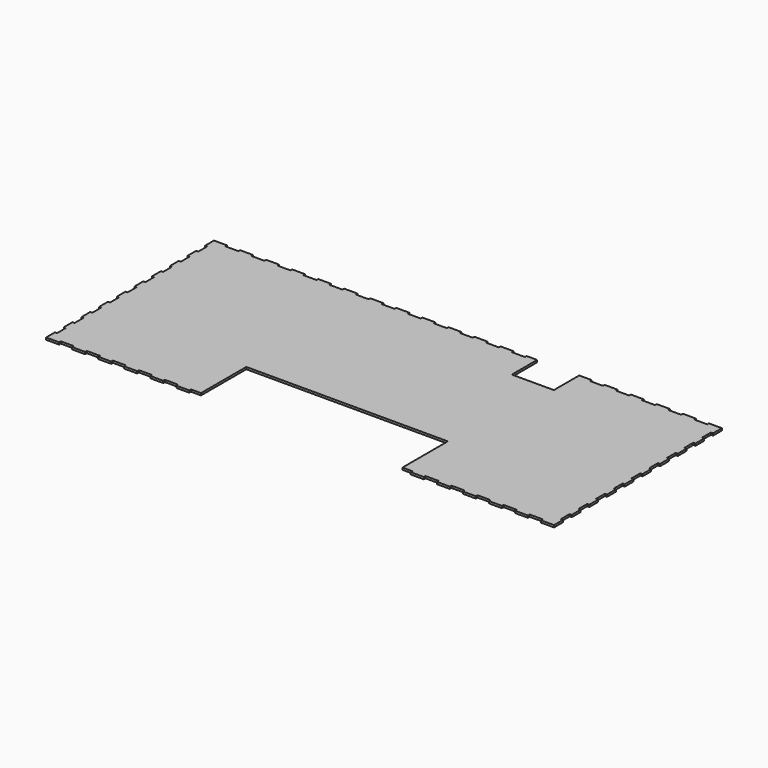
from build123d import *

# Parameters (mm, degrees)
F1_DEPTH = 3.175


# Not quite as in the source:
# - ends of sketch curves that miss each other by under 0.0002 mm in the source are joined
# - a feature names something its author has since deleted; it is built from what else it names


with BuildPart() as f1:
    # F0 (on Top) → F1 (new body)
    with BuildSketch(Plane.XY):
        Polygon((-364.473717838, 158.75), (-384.175, 158.75), (-384.175, 142.039473604), (-381, 142.039473604), (-381, 125.328947208), (-384.175, 125.328947208), (-384.175, 108.618420812), (-381, 108.618420812), (-381, 91.907894416), (-384.175, 91.907894416), (-384.175, 75.19736802), (-381, 75.19736802), (-381, 58.486841624), (-384.175, 58.486841624), (-384.175, 41.776315228), (-381, 41.776315228), (-381, 25.065788832), (-384.175, 25.065788832), (-384.175, 8.355262436), (-381, 8.355262436), (-381, -8.35526396), (-384.175, -8.35526396), (-384.175, -25.065790356), (-381, -25.065790356), (-381, -41.776316752), (-384.175, -41.776316752), (-384.175, -58.486843148), (-381, -58.486843148), (-381, -75.197369544), (-384.175, -75.197369544), (-384.175, -91.90789594), (-381, -91.90789594), (-381, -108.618422336), (-384.175, -108.618422336), (-384.175, -125.328948732), (-381, -125.328948732), (-381, -142.039475128), (-384.175, -142.039475128), (-384.175, -158.750001524), (-381, -158.750001524), (-364.473717838, -158.75), (-364.473717838, -155.575), (-344.772435676, -155.575), (-344.772435676, -158.75), (-325.071153514, -158.75), (-325.071153514, -155.575), (-305.369871352, -155.575), (-305.369871352, -158.75), (-285.66858919, -158.75), (-285.66858919, -155.575), (-265.967307028, -155.575), (-265.967307028, -158.75), (-246.266024866, -158.75), (-246.266024866, -155.575), (-226.564742704, -155.575), (-226.564742704, -158.75), (-206.863460542, -158.75), (-206.863460542, -155.575), (-187.16217838, -155.575), (-187.16217838, -158.75), (-167.460896218, -158.75), (-167.460896218, -155.575), (-152.4, -155.575), (-152.4, -69.85), (152.4, -69.85), (152.4, -155.575), (167.460900536, -155.575), (167.460900536, -158.75), (187.162182698, -158.75), (187.162182698, -155.575), (206.86346486, -155.575), (206.86346486, -158.75), (226.564747022, -158.75), (226.564747022, -155.575), (246.266029184, -155.575), (246.266029184, -158.75), (265.967311346, -158.75), (265.967311346, -155.575), (285.668593508, -155.575), (285.668593508, -158.75), (305.36987567, -158.75), (305.36987567, -155.575), (325.071157832, -155.575), (325.071157832, -158.75), (344.772439994, -158.75), (344.772439994, -155.575), (364.473722156, -155.575), (364.473722156, -158.75), (381, -158.75), (384.175004318, -158.75), (384.175004318, -155.575), (384.175, -142.039475128), (381, -142.039475128), (381, -125.328948732), (384.175, -125.328948732), (384.175, -108.618422336), (381, -108.618422336), (381, -91.90789594), (384.175, -91.90789594), (384.175, -75.197369544), (381, -75.197369544), (381, -58.486843148), (384.175, -58.486843148), (384.175, -41.776316752), (381, -41.776316752), (381, -25.065790356), (384.175, -25.065790356), (384.175, -8.35526396), (381, -8.35526396), (381, 8.355262436), (384.175, 8.355262436), (384.175, 25.065788832), (381, 25.065788832), (381, 41.776315228), (384.175, 41.776315228), (384.175, 58.486841624), (381, 58.486841624), (381, 75.19736802), (384.175, 75.19736802), (384.175, 91.907894416), (381, 91.907894416), (381, 108.618420812), (384.175, 108.618420812), (384.175, 125.328947208), (381, 125.328947208), (381, 142.039473604), (384.175, 142.039473604), (384.175, 158.75), (364.473722156, 158.75), (364.473722156, 155.575), (344.772439994, 155.575), (344.772439994, 158.75), (325.071157832, 158.75), (325.071157832, 155.575), (305.36987567, 155.575), (305.36987567, 158.75), (285.668593508, 158.75), (285.668593508, 155.575), (268.605, 155.575), (265.967311346, 155.575), (265.967311346, 158.75), (246.266029184, 158.75), (246.266029184, 155.575), (226.564747022, 155.575), (226.564747022, 158.75), (206.86346486, 158.75), (206.86346486, 155.575), (187.162182698, 155.575), (187.162182698, 158.75), (168.275, 158.75), (168.275, 110.814742744), (104.775, 110.814742744), (104.775, 158.75), (88.655771888, 158.75), (88.655771888, 155.575), (68.954489726, 155.575), (68.954489726, 158.75), (49.253207564, 158.75), (49.253207564, 155.575), (29.551925402, 155.575), (29.551925402, 158.75), (9.85064324, 158.75), (9.85064324, 155.575), (-9.850638922, 155.575), (-9.850638922, 158.75), (-29.551921084, 158.75), (-29.551921084, 155.575), (-49.253203246, 155.575), (-49.253203246, 158.75), (-68.954485408, 158.75), (-68.954485408, 155.575), (-88.65576757, 155.575), (-88.65576757, 158.75), (-108.357049732, 158.75), (-108.357049732, 155.575), (-128.058331894, 155.575), (-128.058331894, 158.75), (-147.759614056, 158.75), (-147.759614056, 155.575), (-167.460896218, 155.575), (-167.460896218, 158.75), (-187.16217838, 158.75), (-187.16217838, 155.575), (-206.863460542, 155.575), (-206.863460542, 158.75), (-226.564742704, 158.75), (-226.564742704, 155.575), (-246.266024866, 155.575), (-246.266024866, 158.75), (-265.967307028, 158.75), (-265.967307028, 155.575), (-285.66858919, 155.575), (-285.66858919, 158.75), (-305.369871352, 158.75), (-305.369871352, 155.575), (-325.071153514, 155.575), (-325.071153514, 158.75), (-344.772435676, 158.75), (-344.772435676, 155.575), (-364.473717838, 155.575), align=None)
    extrude(amount=F1_DEPTH)


solid = f1.part
